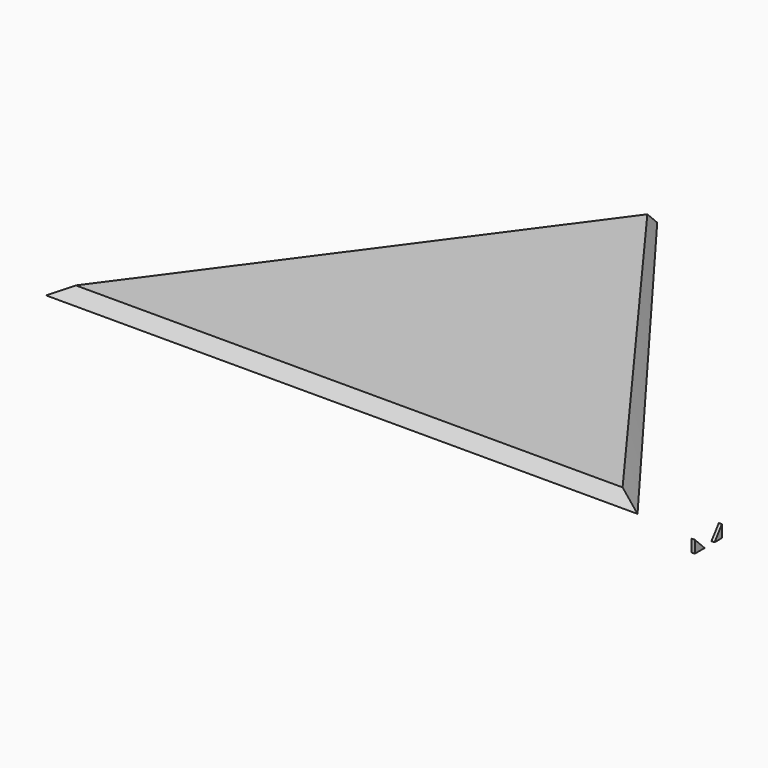
from build123d import *

# Parameters (mm, degrees)
F10_DEPTH = 3.175


# Not quite as in the source:
# - a length typed as a fraction of an inch, garbled in the dataset ("3 / 203.2 mm" for 3/8 in), is restored


with BuildPart() as f7:
    # F6 (on offset) → F7 section 0
    with BuildSketch(Plane.XY.offset(12.7)):
        Polygon((0, 393.7), (-281.7812500119, 9.5249999841), (0, 9.5249999841), (281.7812500119, 9.5249999841), align=None)
    # F1 (on Top) → F7 section 1
    with BuildSketch(Plane.XY):
        Polygon((-304.8, 0), (0, 0), (304.8, 0), (0, 406.4), align=None)
    loft()


with BuildPart() as f10:
    # F9 (on offset) → F10 (new body)
    with BuildSketch(Plane.YZ.offset(381)):
        Polygon((9.5249999841, 0), (9.5249999841, 12.7), (0, 0), align=None)
    extrude(amount=F10_DEPTH)


with BuildPart() as f10b:
    # F9 (on offset) → F10, piece 2 (new body)
    with BuildSketch(Plane.YZ.offset(381)):
        Polygon((-25.4, 0), (-12.7, 0), (-25.4, 12.7), align=None)
    extrude(amount=F10_DEPTH)


solid = Compound([f7.part, f10.part, f10b.part])
